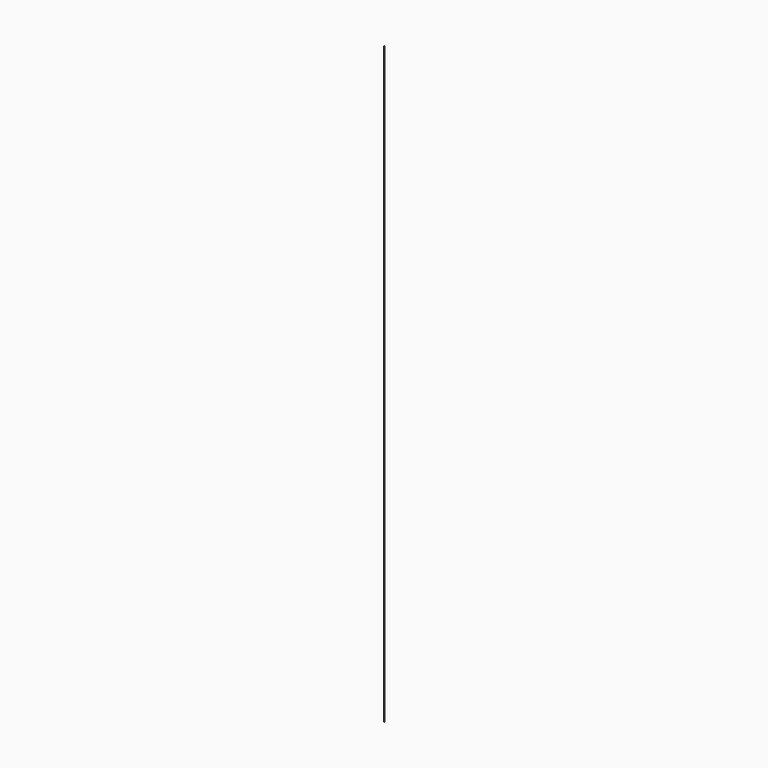
from build123d import *

# Parameters (mm, degrees)
F0_R     = 5.4426660598
F0_R_2   = 8.2339087149
F0_R_3   = 12.9854168842
F1_DEPTH = 500000


with BuildPart() as f1:
    # F0 (on Top) → F1 (new body)
    with BuildSketch(Plane.XY):
        with BuildLine():
            Line((-54.2979964743, 50), (-54.2979964743, 0))
            add(Edge.make_bspline(
                [(-54.2979964743, 0), (-47.3757010279, -9.8194904065), (-40.5416094951, -17.7953065043), (-33.7962601525, -23.9161970139)],
                knots=[0, 0, 0, 0, 19.3575525772, 19.3575525772, 19.3575525772, 19.3575525772], degree=3))
            add(Edge.make_bspline(
                [(-33.7962601525, -23.9161970139), (-29.5866312809, -27.7361144267), (-25.4115652053, -30.833586128), (-21.2711927607, -33.2058773528)],
                knots=[19.3575525772, 19.3575525772, 19.3575525772, 19.3575525772, 31.4381888904, 31.4381888904, 31.4381888904, 31.4381888904], degree=3))
            Line((-21.2711927607, -33.2058773528), (-5.8090212984, -21.7527246851))
            Line((-5.8090212984, -21.7527246851), (10.3962879922, -21.7125103847))
            Line((10.3962879922, -21.7125103847), (21.0729385004, -31.2409453996))
            add(Edge.make_bspline(
                [(21.0729385004, -31.2409453996), (30.142348872, -24.8226587171), (39.0211662161, -14.4205185512), (47.7077388138, 0)],
                knots=[73.8763251974, 73.8763251974, 73.8763251974, 73.8763251974, 102.0057352881, 102.0057352881, 102.0057352881, 102.0057352881], degree=3))
            Line((47.7077388138, 0), (47.7077388138, 50))
            Line((47.7077388138, 50), (16.7225152254, 61.3158904016))
            Line((16.7225152254, 61.3158904016), (-16.2481181324, 65.3482675552))
            Line((-16.2481181324, 65.3482675552), (-54.2979964743, 50))
        make_face()
        Circle(F0_R, mode=Mode.SUBTRACT)
        with Locations((-16.4853166789, 23.3640819788)):
            Circle(F0_R_2, mode=Mode.SUBTRACT)
        with Locations((21.9408869743, 26.447666809)):
            Circle(F0_R_3, mode=Mode.SUBTRACT)
        with BuildLine():
            add(Edge.make_bspline(
                [(-33.7962601525, -23.9161970139), (-29.5866312809, -27.7361144267), (-25.4115652053, -30.833586128), (-21.2711927607, -33.2058773528)],
                knots=[19.3575525772, 19.3575525772, 19.3575525772, 19.3575525772, 31.4381888904, 31.4381888904, 31.4381888904, 31.4381888904], degree=3))
            Line((-33.7962601525, -23.9161970139), (-23.1274297827, -34.580830803))
            Line((-23.1274297827, -34.580830803), (-21.2711927607, -33.2058773528))
        make_face()
        with BuildLine():
            add(Edge.make_bspline(
                [(21.0729385004, -31.2409453996), (30.142348872, -24.8226587171), (39.0211662161, -14.4205185512), (47.7077388138, 0)],
                knots=[73.8763251974, 73.8763251974, 73.8763251974, 73.8763251974, 102.0057352881, 102.0057352881, 102.0057352881, 102.0057352881], degree=3))
            Line((21.0729385004, -31.2409453996), (28.8230053729, -38.1575348767))
            Line((28.8230053729, -38.1575348767), (47.7077388138, 0))
        make_face()
    extrude(amount=F1_DEPTH)


solid = f1.part
